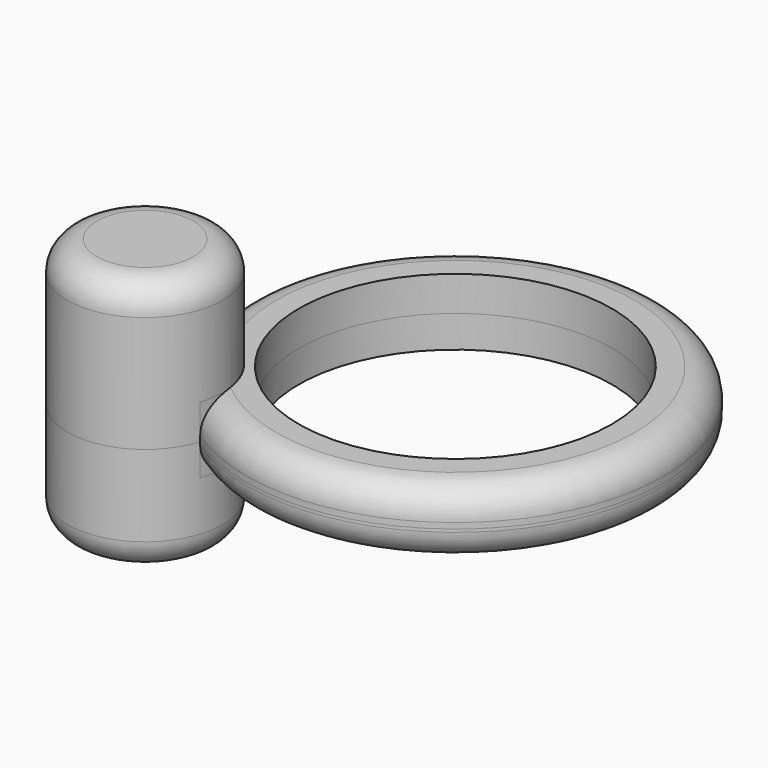
from build123d import *

# Parameters (mm, degrees)
F0_R          = 36.4407990547
F0_R_2        = 27.3961880776
F1_DEPTH      = 6.096
F2_R          = 13.5314507832
F3_DEPTH      = 25.4
F3_DEPTH_BACK = 19.304
F4_R          = 5.08
F5_DEPTH      = 11.684
F6_T4_ANGLE   = 359.64
F6_S5_R       = 13.5314507832
F6_T6_DEPTH   = 57
F6_T10_ANGLE  = 359.64
F6_S11_R      = 13.5314507832
F6_T12_DEPTH  = 57


# Not quite as in the source:
# - a fillet or chamfer that OpenCascade refuses, or shapes differently, is made with other operations: its cross-section is extruded or revolved along the edge and cut away or added


with BuildPart() as f1:
    # F0 (on Top) → F1 (new body)
    with BuildSketch(Plane.XY):
        Circle(F0_R)
        Circle(F0_R_2, mode=Mode.SUBTRACT)
    extrude(amount=F1_DEPTH)

    # F2 (on Top) → F3 (join, two sides)
    with BuildSketch(Plane.XY) as f3_sk:
        with Locations((-33.5037633777, -25.9826220572)):
            Circle(F2_R)
    extrude(amount=F3_DEPTH)
    extrude(f3_sk.sketch, amount=-F3_DEPTH_BACK)

    # F4
    f4_edges = [f1.edges().sort_by_distance(p)[0] for p in [
        (-47.035214, -25.982622, 25.4),
        (-47.035214, -25.982622, -19.304),
    ]]
    fillet(f4_edges, radius=F4_R)

    # F5 (add): a face of the model
    f5_faces = [f1.faces().sort_by_distance(p)[0] for p in [
        (-19.1117163602, -28.201914774, 6.096),
    ]]
    extrude(f5_faces, amount=-F5_DEPTH)

    # F6: fillet of radius 5.08 on 2 edges, made by hand


with BuildPart() as f6_tool2:
    # F6_s3 → F6_t4 (revolve)
    with BuildSketch(Plane(origin=(0, 0, 0), x_dir=(0, 0, 1), z_dir=(0.6103395994, -0.7921398699, 0))):
        with BuildLine():
            ThreePointArc((-0.508, 36.4407990547), (-4.1001024484, 34.9529015031), (-5.588, 31.3607990547))
            Line((-5.588, 31.3607990547), (-5.588, 36.4407990547))
            Line((-5.588, 36.4407990547), (-0.508, 36.4407990547))
        make_face()
    revolve(axis=Axis((0, 0, -5.588), (0, 0, -1)), revolution_arc=F6_T4_ANGLE)

    # F6_s5 → F6_t6 (cut, symmetric)
    with BuildSketch(Plane.XY.offset(-3)):
        with Locations((-33.5037633777, -25.9826220572)):
            Circle(F6_S5_R)
    extrude(amount=F6_T6_DEPTH, both=True, mode=Mode.SUBTRACT)


with BuildPart() as f1_1:
    add(f1.part)

    # F6_t1: cut F6_tool2
    add(f6_tool2.part, mode=Mode.SUBTRACT)


with BuildPart() as f6_tool8:
    # F6_s9 → F6_t10 (revolve)
    with BuildSketch(Plane(origin=(0, 0, 0), x_dir=(0, 0, 1), z_dir=(0.6103395994, -0.7921398699, 0))):
        with BuildLine():
            ThreePointArc((1.016, 36.4407990547), (4.6081024484, 34.9529015031), (6.096, 31.3607990547))
            Line((6.096, 31.3607990547), (6.096, 36.4407990547))
            Line((6.096, 36.4407990547), (1.016, 36.4407990547))
        make_face()
    revolve(axis=Axis((0, 0, 6.096), (0, 0, -1)), revolution_arc=F6_T10_ANGLE)

    # F6_s11 → F6_t12 (cut, symmetric)
    with BuildSketch(Plane.XY.offset(3.6)):
        with Locations((-33.5037633777, -25.9826220572)):
            Circle(F6_S11_R)
    extrude(amount=F6_T12_DEPTH, both=True, mode=Mode.SUBTRACT)


with BuildPart() as f1_2:
    add(f1_1.part)

    # F6_t7: cut F6_tool8
    add(f6_tool8.part, mode=Mode.SUBTRACT)


solid = f1_2.part
